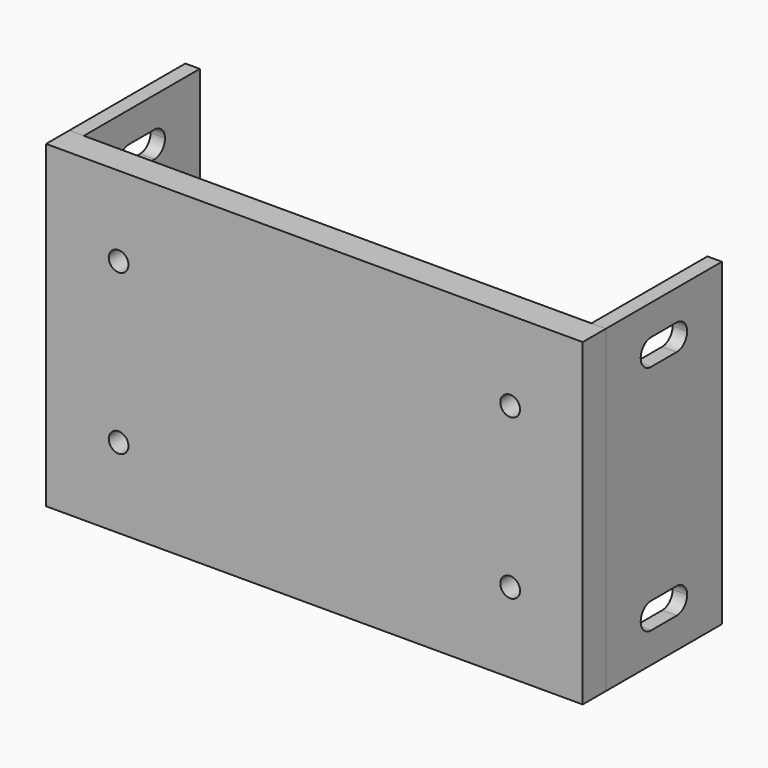
from build123d import *

# Parameters (mm, degrees)
F0_W     = 185
F0_H     = 110
F1_DEPTH = 5
F3_D     = 6.8
F4_W     = 50
F4_H     = 110
F5_DEPTH = 5
F6_W     = 20
F6_H     = 9
F7_DEPTH = 185.001
F8_R     = 4.49999


# Not quite as in the source:
# - a fillet or chamfer is up to 0.001 mm smaller than in the source, because OpenCascade refuses the exact size


with BuildPart() as f1:
    # F0 (on Front) → F1 (new body, symmetric)
    with BuildSketch(Plane.XZ):
        Rectangle(F0_W, F0_H)
    extrude(amount=F1_DEPTH, both=True)

    # F3 (through all)
    with Locations(Plane.XZ.offset(5)):
        with Locations((-67.5, 27.5), (-67.5, -27.5), (67.5, -27.5), (67.5, 27.5)):
            Hole(F3_D / 2)


with BuildPart() as f5:
    # F4 (on face) → F5 (new body)
    with BuildSketch(Plane.YZ.offset(92.5)):
        with Locations((30, 0)):
            Rectangle(F4_W, F4_H)
    extrude(amount=-F5_DEPTH)

    # F6 (on face) → F7 (cut, through all)
    with BuildSketch(Plane.YZ.offset(92.5)):
        with Locations((30, 40)):
            Rectangle(F6_W, F6_H)
        with Locations((30, -40)):
            Rectangle(F6_W, F6_H)
    extrude(amount=-F7_DEPTH, mode=Mode.SUBTRACT)

    # F8 (radius 4.5 in the source; OpenCascade refuses exactly that, so slightly less here)
    f8_edges = [f5.edges().sort_by_distance(p)[0] for p in [
        (90, 20, 35.5),
        (90, 20, 44.5),
        (90, 20, -35.5),
        (90, 20, -44.5),
        (90, 40, -35.5),
        (90, 40, 44.5),
        (90, 40, 35.5),
        (90, 40, -44.5),
    ]]
    fillet(f8_edges, radius=F8_R)


with BuildPart() as f9_1:
    # F9: instance of F5
    add(f5.part.mirror(Plane.YZ))


solid = Compound([f1.part, f5.part, f9_1.part])
